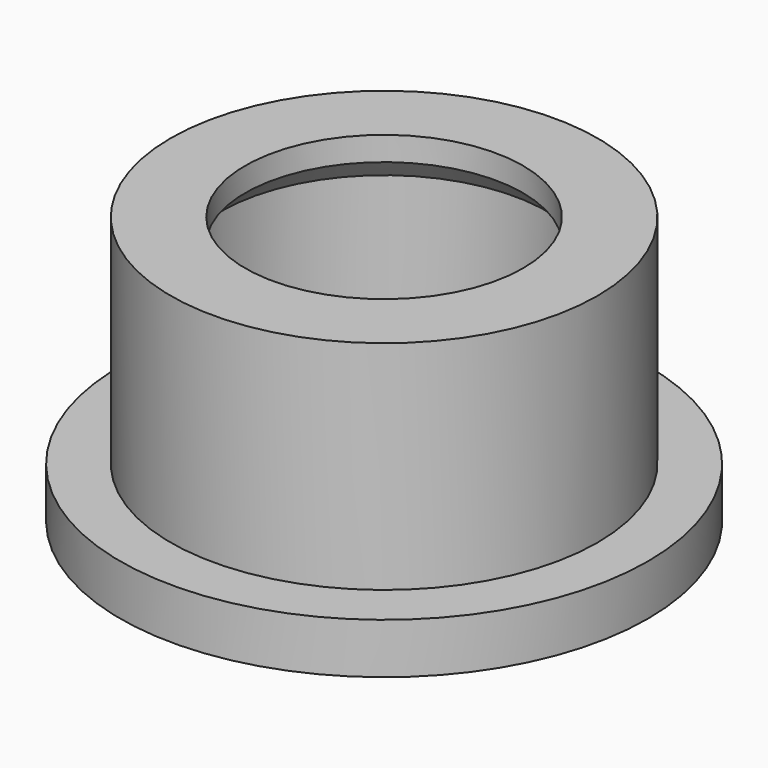
from build123d import *

# Parameters (mm, degrees)
F6_R      = 5.225
F7_DEPTH  = 1
F5_R      = 4.225
F5_R_2    = 3.225
F8_DEPTH  = 4.3
F9_R      = 3.225
F9_R_2    = 2.75
F10_DEPTH = 0.95
F11_SIZE  = 0.47499
F12_SIZE  = 0.475


# Not quite as in the source:
# - a fillet or chamfer is up to 0.001 mm smaller than in the source, because OpenCascade refuses the exact size


with BuildPart() as f7:
    # F6 (on face) → F7 (new body)
    with BuildSketch(Plane.XY):
        Circle(F6_R)
    extrude(amount=-F7_DEPTH)



with BuildPart() as f7b:
    # F5 (on Top) → F7, piece 2 (new body)
    with BuildSketch(Plane.XY):
        Circle(F5_R)
        Circle(F5_R_2, mode=Mode.SUBTRACT)
    extrude(amount=-F7_DEPTH)


with BuildPart() as f7_1:
    add(f7.part)

    add(f7b.part)  # F8 merges F7b
    # F5 (on Top) → F8 (join)
    with BuildSketch(Plane.XY):
        Circle(F5_R)
        Circle(F5_R_2, mode=Mode.SUBTRACT)
    extrude(amount=F8_DEPTH)

    # F9 (on face) → F10 (join)
    with BuildSketch(Plane.XY.offset(4.3)):
        Circle(F9_R)
        Circle(F9_R_2, mode=Mode.SUBTRACT)
    extrude(amount=-F10_DEPTH)

    # F11 (size 0.475 in the source; OpenCascade refuses exactly that, so slightly less here)
    f11_edges = [f7_1.edges().sort_by_distance(p)[0] for p in [
        (-2.75, 0, 3.35),
    ]]
    chamfer(f11_edges, length=F11_SIZE)

    # F12
    f12_edges = [f7_1.edges().sort_by_distance(p)[0] for p in [
        (-3.225, 0, 0),
    ]]
    chamfer(f12_edges, length=F12_SIZE)


solid = f7_1.part
